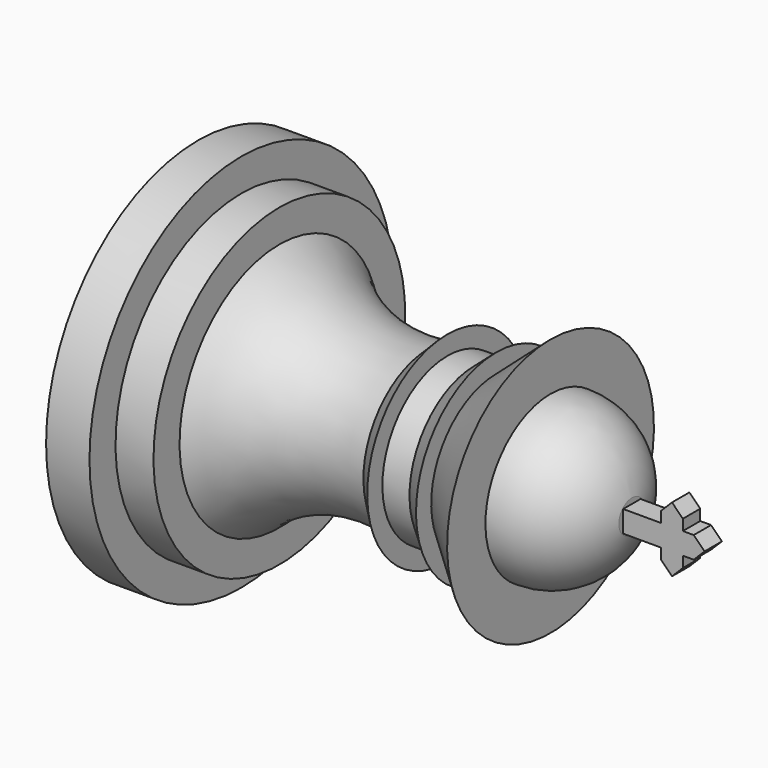
from build123d import *

# Parameters (mm, degrees)
F0_W          = 5.08
F0_H          = 5.08
F2_DEPTH      = 2.54
F2_DEPTH_BACK = 2.54
F3_SIZE2      = 2.53999
F3_SIZE       = 2.53999


# Not quite as in the source:
# - a fillet or chamfer is up to 0.001 mm smaller than in the source, because OpenCascade refuses the exact size


with BuildPart() as f1:
    # F0 (on Front) → F1 (revolve)
    with BuildSketch(Plane.XZ):
        with BuildLine():
            Line((-120.65, 0), (-19.05, 0))
            Line((-19.05, 0), (-19.05, 2.54))
            Line((-19.05, 2.54), (-19.05, 3.81))
            ThreePointArc((-19.05, 3.81), (-25.8165229562, 14.8770320486), (-38.1, 19.0461114431))
            Line((-38.1, 19.0461114431), (-38.1, 30.2734401025))
            Line((-38.1, 30.2734401025), (-50.8, 19.0461114431))
            Line((-50.8, 19.0461114431), (-50.8, 23.4911114431))
            Line((-50.8, 23.4911114431), (-55.88, 19.0461114431))
            Line((-55.88, 19.0461114431), (-62.23, 19.0461114431))
            Line((-62.23, 19.0461114431), (-62.23, 23.4911114431))
            Line((-62.23, 23.4911114431), (-66.675, 19.0461114431))
            ThreePointArc((-66.675, 19.0461114431), (-85.4281931482, 19.6893537461), (-101.6, 29.2061114431))
            Line((-101.6, 29.2061114431), (-101.6, 36.83))
            Line((-101.6, 36.83), (-110.49, 36.83))
            Line((-110.49, 36.83), (-110.49, 44.45))
            Line((-110.49, 44.45), (-120.65, 44.45))
            Line((-120.65, 44.45), (-120.65, 0))
        make_face()
    revolve(axis=Axis((-69.85, 0, 0), (-1, 0, 0)))

    # F0 (on Front) → F2 (join, two sides)
    with BuildSketch(Plane.XZ) as f2_sk:
        with Locations((-2.54, 0)):
            Rectangle(F0_W, F0_H)
        with Locations((-7.62, -5.08)):
            Rectangle(F0_W, F0_H)
        with Locations((-7.62, 0)):
            Rectangle(F0_W, F0_H)
        with Locations((-7.62, 5.08)):
            Rectangle(F0_W, F0_H)
        Polygon((-19.05, 2.54), (-19.05, 0), (-19.05, -2.54), (-10.16, -2.54), (-10.16, 2.54), align=None)
    extrude(amount=F2_DEPTH)
    extrude(f2_sk.sketch, amount=-F2_DEPTH_BACK)

    # F3 (size 2.54 and 2.54 in the source; OpenCascade refuses exactly that, so slightly less here)
    f3_edges = [f1.edges().sort_by_distance(p)[0] for p in [
        (-10.16, 0, 7.62),
        (-5.08, 0, 7.62),
        (0, 0, 2.54),
        (0, 0, -2.54),
        (-5.08, 0, -7.62),
        (-10.16, 0, -7.62),
    ]]
    chamfer(f3_edges, length=F3_SIZE, length2=F3_SIZE2)


solid = f1.part
